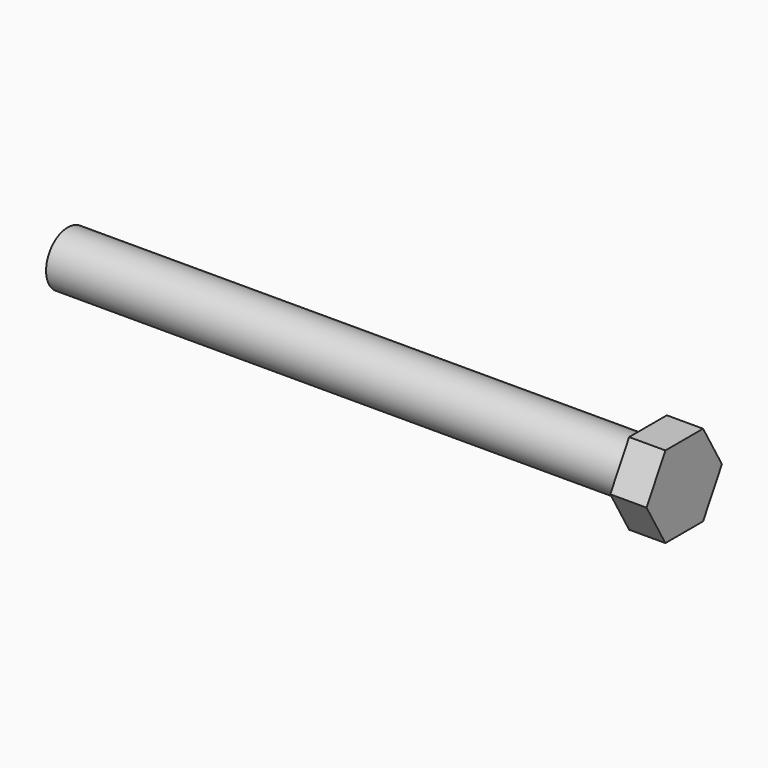
from build123d import *

# Parameters (mm, degrees)
F1_DEPTH = 6.35
F2_R     = 4.7625
F3_DEPTH = 101.6


# Not quite as in the source:
# - a length typed as a fraction of an inch, garbled in the dataset ("3 / 203.2 mm" for 3/8 in), is restored


with BuildPart() as f1:
    # F0 (on Right) → F1 (new body)
    with BuildSketch(Plane.YZ):
        Polygon((4.1244459855, 7.14375), (-4.1244459855, 7.14375), (-8.248891971, 0), (-4.1244459855, -7.14375), (4.1244459855, -7.14375), (8.248891971, 0), align=None)
    extrude(amount=F1_DEPTH)

    # F2 (on Right) → F3 (join)
    with BuildSketch(Plane.YZ):
        Circle(F2_R)
    extrude(amount=-F3_DEPTH)


solid = f1.part
